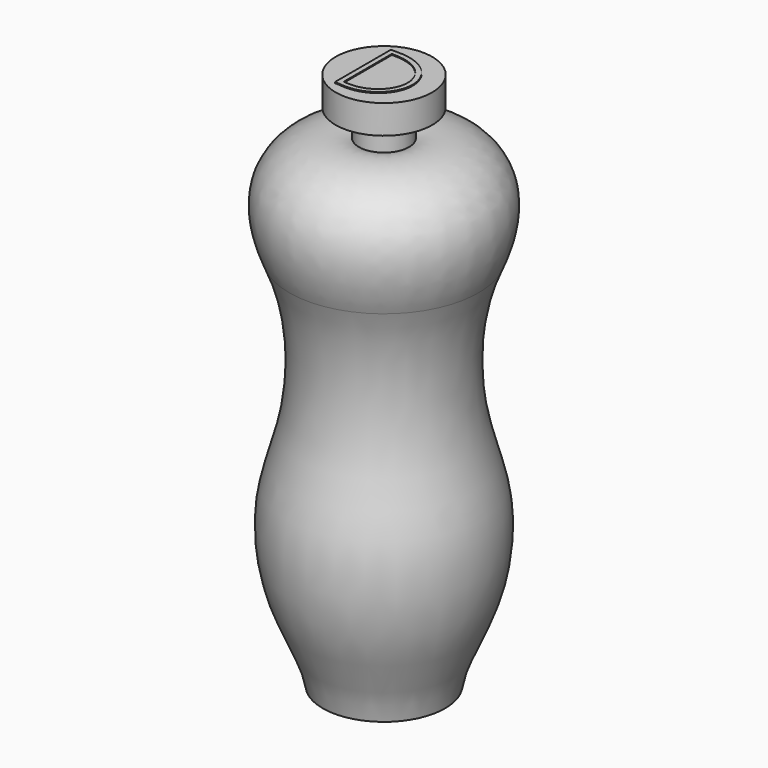
from build123d import *

# Parameters (mm, degrees)
F3_DEPTH = 0.254


# Not quite as in the source:
# - the dataset's text gives a spline's control points without its knots; the knots are read off the source's solid


with BuildPart() as f1:
    # F0 (on Front) → F1 (revolve)
    with BuildSketch(Plane.XZ):
        with BuildLine():
            add(Edge.make_bspline(
                [(-24.00300093, 34.1219119728), (-34.5925595611, 58.8308796287), (-12.001500465, 64.243324101), (-6.3537359238, 60.9487965703)],
                knots=[0, 0, 0, 0, 32.1119649425, 32.1119649425, 32.1119649425, 32.1119649425], degree=3))
            add(Edge.make_bspline(
                [(-24.00300093, 34.1219119728), (-18.9536922311, 22.7837625244), (-18.5681374824, -0.2470894327), (-26.8785367938, -18.6238056214), (-24.691088195, -42.1466133195), (-16.1825619965, -55.7671880803), (-15.5313527212, -61.4194460213)],
                knots=[0.203666813, 0.203666813, 0.203666813, 0.203666813, 0.4410776761, 0.6217292798, 0.8149119798, 1, 1, 1, 1], degree=3))
            Line((-15.5313527212, -61.4194460213), (0, -61.4194460213))
            Line((0, -61.4194460213), (0, 75.068205595))
            Line((0, 75.068205595), (-12.2368233278, 75.068205595))
            Line((-12.2368233278, 75.068205595), (-12.2368233278, 67.7731782198))
            Line((-12.2368233278, 67.7731782198), (-6.3537359238, 67.7731782198))
            Line((-6.3537359238, 67.7731782198), (-6.3537359238, 60.9487965703))
        make_face()
    revolve(axis=Axis((0, 0, 6.8243797868), (0, 0, -1)))


with BuildPart() as f3:
    # F2 (on face) → F3 (new body)
    with BuildSketch(Plane.XY.offset(75.068205595)):
        with BuildLine():
            add(Edge.make_bspline(
                [(-4.062971086, 8.8058835483), (-2.1933640147, 8.8714837532), (1.157297254, 8.386143894), (4.8815568375, 6.1718222853), (6.7372592969, 3.4796927349), (7.4115294482, 1.0933105566), (7.5036193193, -0.7473994059), (7.1702119433, -2.5600192903), (6.4470817235, -4.2581784287), (5.3703358944, -5.7927542709), (3.5050178222, -7.5465765347), (0.4402015685, -9.0509652568), (-2.5993347226, -9.2105905441), (-4.2094985396, -8.9655655025)],
                knots=[0, 0, 0, 0, 0.125, 0.25, 0.375, 0.4375, 0.5, 0.5625, 0.625, 0.6875, 0.75, 0.875, 1, 1, 1, 1], degree=3))
            Line((-4.062971086, 8.8058835483), (-5.2884371173, 8.8058835483))
            Line((-5.2884371173, 8.8058835483), (-5.2884371173, 7.5366646051))
            Line((-5.2884371173, 7.5366646051), (-5.2884371173, -7.7100195922))
            Line((-5.2884371173, -7.7100195922), (-5.2884371173, -8.9655655025))
            Line((-5.2884371173, -8.9655655025), (-4.2094985396, -8.9655655025))
        make_face()
        with BuildLine():
            Line((-4.0184371173, -7.7100195922), (-4.0184371173, 7.5366646051))
            add(Edge.make_bspline(
                [(-4.0184371173, 7.5366646051), (3.0470998026, 7.7845780179), (9.9553181322, -1.0778744554), (1.6835748684, -8.5777174681), (-4.0184371173, -7.7100195922)],
                knots=[0, 0, 0, 0, 0.509491159, 1, 1, 1, 1], degree=3))
        make_face(mode=Mode.SUBTRACT)
    extrude(amount=F3_DEPTH)


solid = Compound([f1.part, f3.part])
